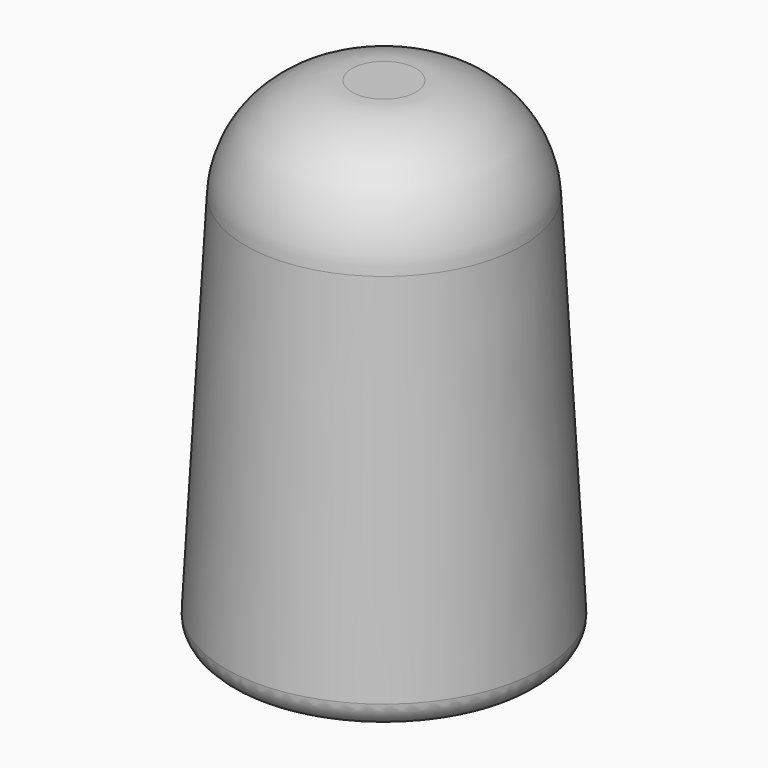
from build123d import *

# Parameters (mm, degrees)
F2_R = 1.99999
F3_R = 9


# Not quite as in the source:
# - a fillet or chamfer is up to 0.001 mm smaller than in the source, because OpenCascade refuses the exact size


with BuildPart() as f1:
    # F0 (on Front) → F1 (revolve)
    with BuildSketch(Plane.XZ):
        Polygon((-9.5, -13.2402114049), (-7.5, 23.7597885951), (0, 23.7597885951), (0, 28.8208965212), (-11.5044763215, 28.8208965212), (-11.5044763215, 23.7850059011), (-13.4568578627, -12.3340526108), align=None)
    revolve(axis=Axis((0, 0, 3.3093634993), (0, 0, -1)))

    # F2 (radius 2 in the source; OpenCascade refuses exactly that, so slightly less here)
    f2_edges = [f1.edges().sort_by_distance(p)[0] for p in [
        (9.5, 0, -13.240211),
        (13.456858, 0, -12.334053),
    ]]
    fillet(f2_edges, radius=F2_R)

    # F3
    f3_edges = [f1.edges().sort_by_distance(p)[0] for p in [
        (11.504476, 0, 28.820897),
    ]]
    fillet(f3_edges, radius=F3_R)


solid = f1.part
